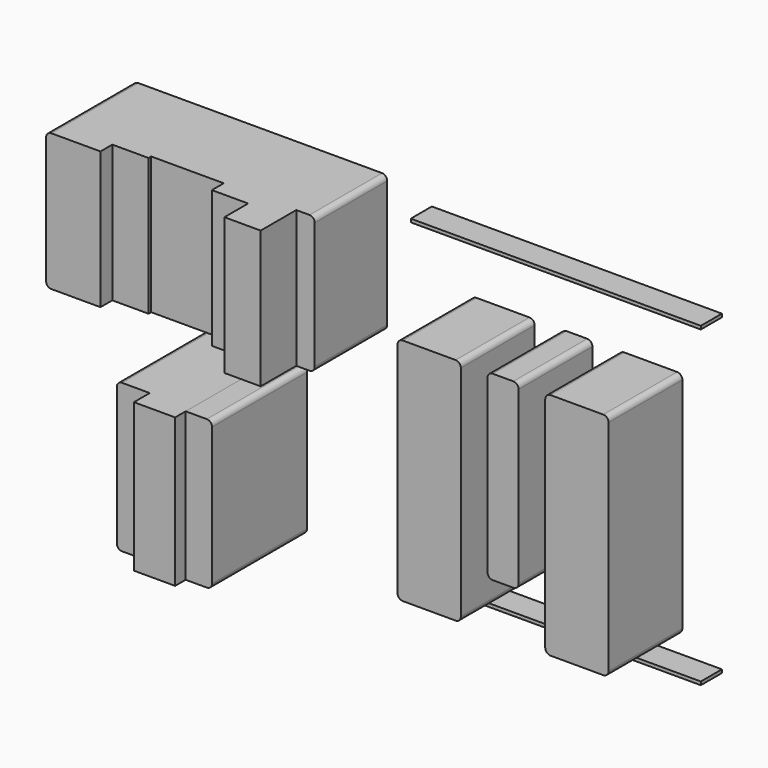
from build123d import *

# Parameters (mm, degrees)
F0_W      = 60.96
F0_H      = 220.98
F1_DEPTH  = 88.9
F0_W_2    = 29.972
F0_H_2    = 175.006
F2_R      = 5.08
F2_2_R    = 5.08
F2_3_R    = 5.08
F3_R      = 5.08
F0_W_3    = 52.3875
F0_H_3    = 132.08
F4_DEPTH  = 104.775
F0_W_4    = 34.925
F5_DEPTH  = 90.5002
F0_W_5    = 69.85
F6_DEPTH  = 87.3252
F7_DEPTH  = 101.6
F8_DEPTH  = 130.175
F0_W_6    = 17.78
F9_DEPTH  = 87.3252
F0_W_7    = 31.75
F0_H_4    = 142.875
F10_DEPTH = 107.95
F0_W_8    = 39.6875
F11_DEPTH = 127
F0_W_9    = 25.4
F12_DEPTH = 114.3
F13_W     = 279.4
F13_H     = 3.175
F14_DEPTH = 25.4
F15_R     = 5.08
F15_2_R   = 5.08
F15_3_R   = 5.08


with BuildPart() as f1:
    # F0 (on Front) → F1 (new body)
    with BuildSketch(Plane.XZ):
        with Locations((432.5366, -250.19)):
            Rectangle(F0_W, F0_H)
    extrude(amount=F1_DEPTH)

    # F2
    f2_edges = [f1.edges().sort_by_distance(p)[0] for p in [
        (463.0166, -44.45, -139.7),
        (402.0566, -44.45, -139.7),
        (402.0566, -44.45, -360.68),
        (463.0166, -44.45, -360.68),
    ]]
    fillet(f2_edges, radius=F2_R)


with BuildPart() as f1b:
    # F0 (on Front) → F1, piece 2 (new body)
    with BuildSketch(Plane.XZ):
        with Locations((574.7766, -250.19)):
            Rectangle(F0_W, F0_H)
    extrude(amount=F1_DEPTH)

    # F2#2
    f2_2_edges = [f1b.edges().sort_by_distance(p)[0] for p in [
        (605.2566, -44.45, -139.7),
        (544.2966, -44.45, -139.7),
        (544.2966, -44.45, -360.68),
        (605.2566, -44.45, -360.68),
    ]]
    fillet(f2_2_edges, radius=F2_2_R)


with BuildPart() as f1c:
    # F0 (on Front) → F1, piece 3 (new body)
    with BuildSketch(Plane.XZ):
        with Locations((503.6566, -227.203)):
            Rectangle(F0_W_2, F0_H_2)
    extrude(amount=F1_DEPTH)

    # F2#3
    f2_3_edges = [f1c.edges().sort_by_distance(p)[0] for p in [
        (518.6426, -44.45, -139.7),
        (488.6706, -44.45, -314.706),
        (518.6426, -44.45, -314.706),
    ]]
    fillet(f2_3_edges, radius=F2_3_R)

    # F3
    f3_edges = [f1c.edges().sort_by_distance(p)[0] for p in [
        (488.6706, -44.45, -139.7),
    ]]
    fillet(f3_edges, radius=F3_R)


with BuildPart() as f4:
    # F0 (on Front) → F4 (new body)
    with BuildSketch(Plane.XZ):
        with Locations((102.39375, -129.54)):
            Rectangle(F0_W_3, F0_H_3)
    extrude(amount=F4_DEPTH)

    # F0 (on Front) → F5 (join)
    with BuildSketch(Plane.XZ):
        with Locations((146.05, -129.54)):
            Rectangle(F0_W_4, F0_H_3)
    extrude(amount=F5_DEPTH)

    # F0 (on Front) → F6 (join)
    with BuildSketch(Plane.XZ):
        with Locations((198.4375, -129.54)):
            Rectangle(F0_W_5, F0_H_3)
    extrude(amount=F6_DEPTH)

    # F0 (on Front) → F7 (join)
    with BuildSketch(Plane.XZ):
        with Locations((250.825, -129.54)):
            Rectangle(F0_W_4, F0_H_3)
    extrude(amount=F7_DEPTH)

    # F0 (on Front) → F8 (join)
    with BuildSketch(Plane.XZ):
        with Locations((285.75, -129.54)):
            Rectangle(F0_W_4, F0_H_3)
    extrude(amount=F8_DEPTH)

    # F0 (on Front) → F9 (join)
    with BuildSketch(Plane.XZ):
        with Locations((312.1025, -129.54)):
            Rectangle(F0_W_6, F0_H_3)
    extrude(amount=F9_DEPTH)

    # F15
    f15_edges = [f4.edges().sort_by_distance(p)[0] for p in [
        (320.9925, -43.6626, -63.5),
        (76.2, -52.3875, -63.5),
        (320.9925, -43.6626, -195.58),
        (76.2, -52.3875, -195.58),
    ]]
    fillet(f15_edges, radius=F15_R)


with BuildPart() as f10:
    # F0 (on Front) → F10 (new body)
    with BuildSketch(Plane.XZ):
        with Locations((162.7124, -322.2625)):
            Rectangle(F0_W_7, F0_H_4)
    extrude(amount=F10_DEPTH)

    # F0 (on Front) → F11 (join)
    with BuildSketch(Plane.XZ):
        with Locations((198.43115, -322.2625)):
            Rectangle(F0_W_8, F0_H_4)
    extrude(amount=F11_DEPTH)

    # F15#2
    f15_2_edges = [f10.edges().sort_by_distance(p)[0] for p in [
        (146.8374, -53.975, -250.825),
        (146.8374, -53.975, -393.7),
    ]]
    fillet(f15_2_edges, radius=F15_2_R)


with BuildPart() as f12:
    # F0 (on Front) → F12 (new body)
    with BuildSketch(Plane.XZ):
        with Locations((230.9749, -322.2625)):
            Rectangle(F0_W_9, F0_H_4)
    extrude(amount=F12_DEPTH)

    # F15#3
    f15_3_edges = [f12.edges().sort_by_distance(p)[0] for p in [
        (243.6749, -57.15, -250.825),
        (243.6749, -57.15, -393.7),
    ]]
    fillet(f15_3_edges, radius=F15_3_R)


with BuildPart() as f14:
    # F13 (on Front) → F14 (new body)
    with BuildSketch(Plane.XZ):
        with Locations((503.6566, -77.7875)):
            Rectangle(F13_W, F13_H)
    extrude(amount=F14_DEPTH)


with BuildPart() as f14b:
    # F13 (on Front) → F14, piece 2 (new body)
    with BuildSketch(Plane.XZ):
        with Locations((503.6566, -379.4125)):
            Rectangle(F13_W, F13_H)
    extrude(amount=F14_DEPTH)


solid = Compound([f1.part, f1b.part, f1c.part, f4.part, f10.part, f12.part, f14.part, f14b.part])
